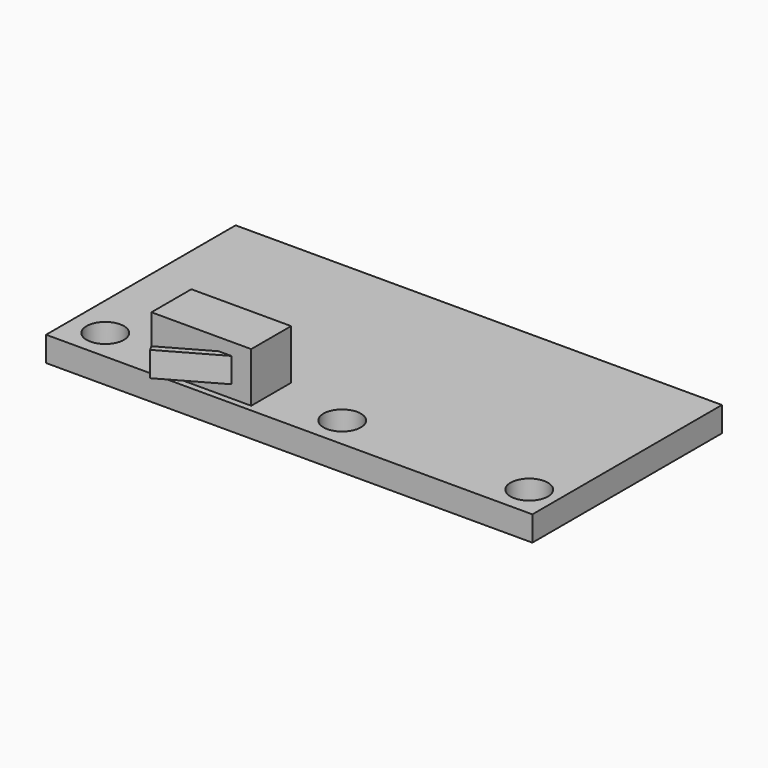
from build123d import *

# Parameters (mm, degrees)
F0_W     = 39
F0_H     = 19
F0_R     = 1.5
F1_DEPTH = 2
F2_W     = 8
F2_H     = 4
F3_DEPTH = 4
F6_DEPTH = 2


with BuildPart() as f1:
    # F0 (on Top) → F1 (new body)
    with BuildSketch(Plane.XY):
        with Locations((19.5, 9.5)):
            Rectangle(F0_W, F0_H)
        with Locations((2.7466891247, 2.5)):
            Circle(F0_R, mode=Mode.SUBTRACT)
        with Locations((21.7466891247, 2.5)):
            Circle(F0_R, mode=Mode.SUBTRACT)
        with Locations((36.7466891247, 2.5)):
            Circle(F0_R, mode=Mode.SUBTRACT)
    extrude(amount=F1_DEPTH)

    # F2 (on face) → F3 (join)
    with BuildSketch(Plane.XY.offset(2)):
        with Locations((12.0512238369, 2.5)):
            Rectangle(F2_W, F2_H)
    extrude(amount=F3_DEPTH)

    # F5 (on face) → F6 (join)
    with BuildSketch(Plane.XY.offset(5)):
        Polygon((15.1900717236, 0.915290064), (14.9440382274, 1.3505687319), (9.7206942123, -1.6018332224), (9.9667277085, -2.0371118903), align=None)
    extrude(amount=-F6_DEPTH)


solid = f1.part
